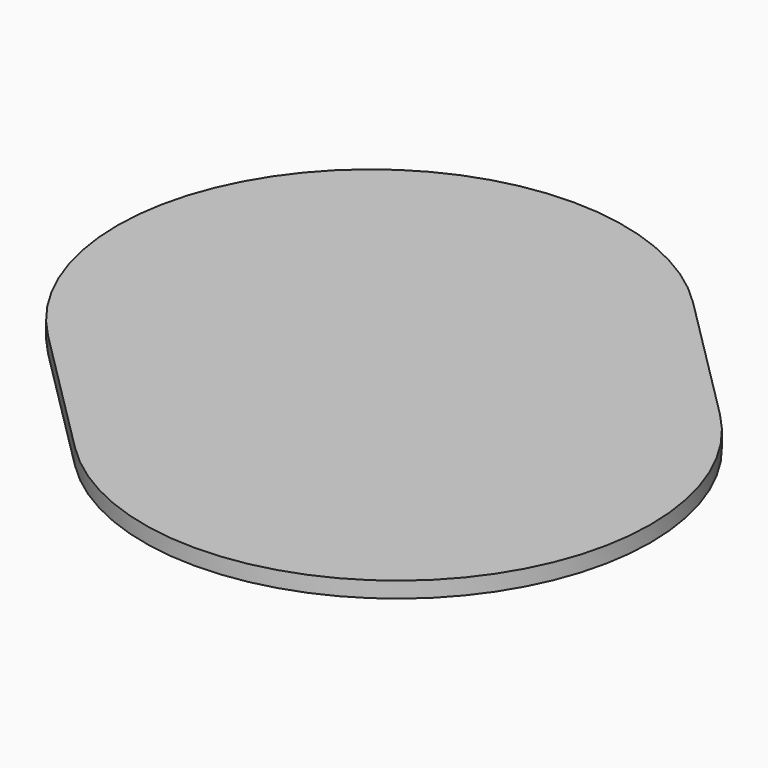
from build123d import *

# Parameters (mm, degrees)
F1_DEPTH = 12.7


# Not quite as in the source:
# - ends of sketch curves that miss each other by under 0.0002 mm in the source are joined


with BuildPart() as f1:
    # F0 (on Top) → F1 (new body)
    with BuildSketch(Plane.XY):
        with BuildLine():
            Line((-5143.3005338, 787.4531622), (-5251.0636914, 895.2161674))
            ThreePointArc((-5251.0636914, 895.2161674), (-5538.4318809371, 895.2161483371), (-5538.4318936371, 607.8479651629))
            Line((-5538.4318936371, 607.8479651629), (-5430.6687424, 500.0849536))
            ThreePointArc((-5430.6687424, 500.0849536), (-5143.3005274629, 500.0849472629), (-5143.3005338, 787.4531622))
        make_face()
    extrude(amount=F1_DEPTH)


solid = f1.part
